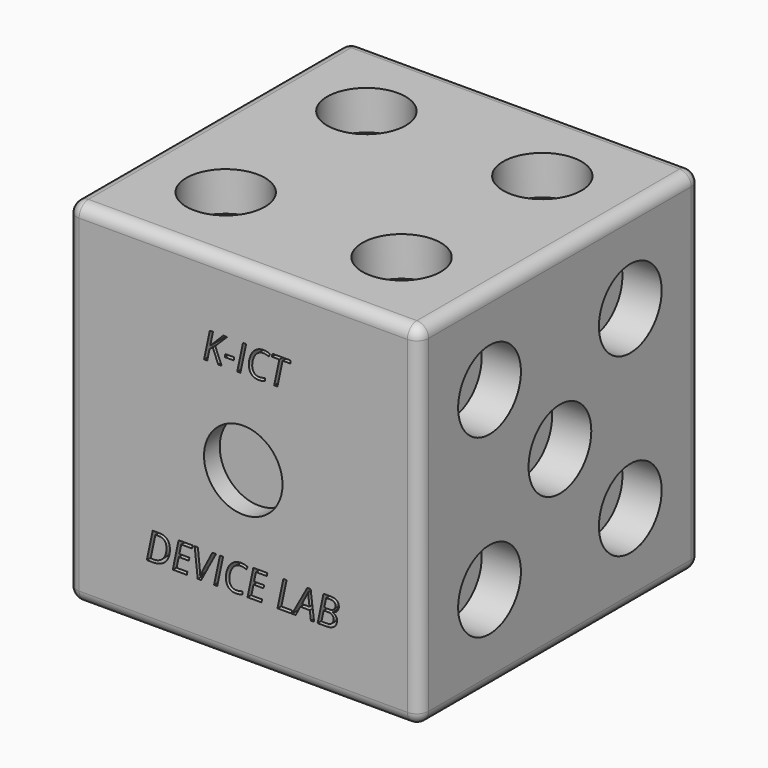
from build123d import *

# Parameters (mm, degrees)
F0_W            = 89.6702081584
F0_H            = 89.6702081584
F1_DEPTH        = 89.67
F2_R            = 10
F3_DEPTH        = 5
F4_R            = 10
F5_DEPTH        = 10
F6_R            = 10
F7_DEPTH        = 10
F8_R            = 10
F9_DEPTH        = 10
F10_R           = 10
F11_DEPTH       = 10
F12_R           = 10
F13_DEPTH       = 10
F14_R           = 3
F15_TEXT_SIZE   = 9.7222222222
F16_DEPTH       = 10
F17_TEXT_SIZE   = 9.9301784329
F17_TEXT_SIZE_2 = 9.7222222222
F18_DEPTH       = 10


# Not quite as in the source:
# - Text() gives the source's letters only with a copy of the font that has no kerning and outlines rounded to 1/6400 em; it was checked with that copy


with BuildPart() as f1:
    # F0 (on Top) → F1 (new body)
    with BuildSketch(Plane.XY):
        Rectangle(F0_W, F0_H)
    extrude(amount=F1_DEPTH)

    # F2 (on face) → F3 (cut)
    with BuildSketch(Plane.XZ.offset(44.8351040792)):
        with Locations((0, 43.7255501747)):
            Circle(F2_R)
    extrude(amount=-F3_DEPTH, mode=Mode.SUBTRACT)

    # F4 (on Top) → F5 (cut)
    with BuildSketch(Plane.XY):
        with Locations((-22.4175520396, -22.4175520396)):
            Circle(F4_R)
        with Locations((22.4175520396, -22.4175520396)):
            Circle(F4_R)
        with Locations((-22.4175520396, 22.4175520396)):
            Circle(F4_R)
        with Locations((22.4175520396, 22.4175520396)):
            Circle(F4_R)
    extrude(amount=F5_DEPTH, mode=Mode.SUBTRACT)

    # F6 (on face) → F7 (cut)
    with BuildSketch(Plane.YZ.offset(44.8351040792)):
        with Locations((-22.4175520396, 67.2525)):
            Circle(F6_R)
        with Locations((22.4175520396, 67.2525)):
            Circle(F6_R)
        with Locations((0, 44.835)):
            Circle(F6_R)
        with Locations((-22.4175520396, 22.4175)):
            Circle(F6_R)
        with Locations((22.4175520396, 22.4175)):
            Circle(F6_R)
    extrude(amount=-F7_DEPTH, mode=Mode.SUBTRACT)

    # F8 (on face) → F9 (cut)
    with BuildSketch(Plane(origin=(-44.8351040792, 0, 0), x_dir=(0, -1, 0), z_dir=(-1, 0, 0))):
        with Locations((0, 44.835)):
            Circle(F8_R)
        with Locations((-22.4175520396, 22.4175)):
            Circle(F8_R)
        with Locations((22.4175520396, 67.2525)):
            Circle(F8_R)
    extrude(amount=-F9_DEPTH, mode=Mode.SUBTRACT)

    # F10 (on face) → F11 (cut)
    with BuildSketch(Plane.XY.offset(89.67)):
        with Locations((22.4175520396, -22.4175520396)):
            Circle(F10_R)
        with Locations((-22.4175520396, -22.4175520396)):
            Circle(F10_R)
        with Locations((22.4175520396, 22.4175520396)):
            Circle(F10_R)
        with Locations((-22.4175520396, 22.4175520396)):
            Circle(F10_R)
    extrude(amount=-F11_DEPTH, mode=Mode.SUBTRACT)

    # F12 (on face) → F13 (cut)
    with BuildSketch(Plane(origin=(0, 44.8351040792, 0), x_dir=(-1, 0, 0), z_dir=(0, 1, 0))):
        with Locations((0, 67.2525)):
            Circle(F12_R)
        with BuildLine():
            ThreePointArc((24.3319919357, 76.546814548), (22.4049782879, 58.9790641618), (38.0219400495, 67.2525))
            ThreePointArc((38.0219400495, 67.2525), (33.6389018111, 75.5259358382), (24.3319919357, 76.546814548))
        make_face()
        with BuildLine():
            ThreePointArc((-24.3319919357, 76.546814548), (-36.2953758877, 61.6355382384), (-18.0219400495, 67.2525))
            ThreePointArc((-18.0219400495, 67.2525), (-19.7485042113, 72.8694617616), (-24.3319919357, 76.546814548))
        make_face()
        with Locations((28.0219400495, 22.4175)):
            Circle(F12_R)
        with Locations((0, 22.4175)):
            Circle(F12_R)
        with Locations((-28.0219400495, 22.4175)):
            Circle(F12_R)
    extrude(amount=-F13_DEPTH, mode=Mode.SUBTRACT)

    # F14
    f14_edges = [f1.edges().sort_by_distance(p)[0] for p in [
        (-44.835104, 0, 0),
        (0, -44.835104, 0),
        (44.835104, 0, 0),
        (0, 44.835104, 0),
        (-44.835104, -44.835104, 44.835),
        (-44.835104, 44.835104, 44.835),
        (44.835104, -44.835104, 44.835),
        (0, -44.835104, 89.67),
        (-44.835104, 0, 89.67),
        (44.835104, 44.835104, 44.835),
        (0, 44.835104, 89.67),
        (44.835104, 0, 89.67),
    ]]
    fillet(f14_edges, radius=F14_R)

    # F15 (on face) → F16 (cut)
    with BuildSketch(Plane(origin=(0, 44.8351040792, 0), x_dir=(-1, 0, 0), z_dir=(0, 1, 0))):
        with Locations((-33.474255372, 41.4943924401)):
            Text('LEE KYONG HEE', F15_TEXT_SIZE, font='Open Sans', font_style=FontStyle.ITALIC, text_align=(TextAlign.LEFT, TextAlign.BOTTOM))
    extrude(amount=-F16_DEPTH, mode=Mode.SUBTRACT)

    # F17 (on face) → F18 (cut)
    with BuildSketch(Plane.XZ.offset(44.8351040792)):
        with Locations((-25, 15.5647751461)):
            Text('DEVICE LAB', F17_TEXT_SIZE, font='Open Sans', font_style=FontStyle.ITALIC, text_align=(TextAlign.LEFT, TextAlign.BOTTOM))
        with Locations((-10.3995466953, 65.3328746557)):
            Text('K-ICT', F17_TEXT_SIZE_2, font='Open Sans', font_style=FontStyle.ITALIC, text_align=(TextAlign.LEFT, TextAlign.BOTTOM))
    extrude(amount=-F18_DEPTH, mode=Mode.SUBTRACT)


solid = f1.part
